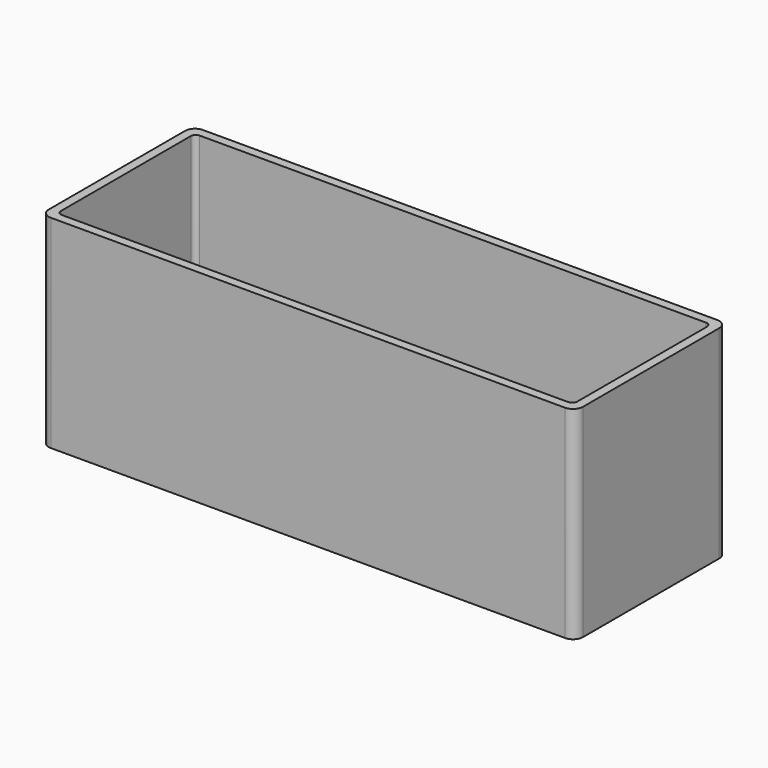
from build123d import *

# Parameters (mm, degrees)
F1_DEPTH = 40.64
F3_DEPTH = 38.608
F5_DEPTH = 4.7752
F6_R     = 1.35255
F7_DEPTH = 4.7752


# Not quite as in the source:
# - a feature names something its author has since deleted; it is built from what else it names


with BuildPart() as f1:
    # F0 (on Top) → F1 (new body)
    with BuildSketch(Plane.XY):
        with BuildLine():
            ThreePointArc((0, 2), (0.5857864376, 0.5857864376), (2, 0))
            Line((2, 0), (105.061, 0))
            ThreePointArc((105.061, 0), (106.4752135624, 0.5857864376), (107.061, 2))
            Line((107.061, 2), (107.061, 36.1))
            ThreePointArc((107.061, 36.1), (106.4752135624, 37.5142135624), (105.061, 38.1))
            Line((105.061, 38.1), (2, 38.1))
            ThreePointArc((2, 38.1), (0.5857864376, 37.5142135624), (0, 36.1))
            Line((0, 36.1), (0, 2))
        make_face()
    extrude(amount=F1_DEPTH)

    # F2 (on face) → F3 (cut)
    with BuildSketch(Plane.XY.offset(40.64)):
        with BuildLine():
            Line((104.261, 36.3), (2.8, 36.3))
            ThreePointArc((2.8, 36.3), (2.0928932188, 36.0071067812), (1.8, 35.3))
            Line((1.8, 35.3), (1.8, 2.8))
            ThreePointArc((1.8, 2.8), (2.0928932188, 2.0928932188), (2.8, 1.8))
            Line((2.8, 1.8), (104.261, 1.8))
            ThreePointArc((104.261, 1.8), (104.9681067812, 2.0928932188), (105.261, 2.8))
            Line((105.261, 2.8), (105.261, 35.3))
            ThreePointArc((105.261, 35.3), (104.9681067812, 36.0071067812), (104.261, 36.3))
        make_face()
    extrude(amount=-F3_DEPTH, mode=Mode.SUBTRACT)

    # F4 (on face) → F5 (join)
    with BuildSketch(Plane(origin=(0, 0, 0), x_dir=(1, 0, 0), z_dir=(0, 0, -1))):
        with BuildLine():
            ThreePointArc((107.061, -2), (106.4752135624, -0.5857864376), (105.061, 0))
            Line((105.061, 0), (101.251, 0))
            Line((101.251, 0), (101.251, -2))
            ThreePointArc((101.251, -2), (102.3669231637, -4.6940768363), (105.061, -5.81))
            Line((105.061, -5.81), (107.061, -5.81))
            Line((107.061, -5.81), (107.061, -2))
        make_face()
        with BuildLine():
            Line((101.251, -36.1), (101.251, -38.1))
            Line((101.251, -38.1), (105.061, -38.1))
            ThreePointArc((105.061, -38.1), (106.4752135624, -37.5142135624), (107.061, -36.1))
            Line((107.061, -36.1), (107.061, -32.29))
            Line((107.061, -32.29), (105.061, -32.29))
            ThreePointArc((105.061, -32.29), (102.3669231637, -33.4059231637), (101.251, -36.1))
        make_face()
        with BuildLine():
            ThreePointArc((5.81, -36.1), (4.6940768363, -33.4059231637), (2, -32.29))
            Line((2, -32.29), (0, -32.29))
            Line((0, -32.29), (0, -36.1))
            ThreePointArc((0, -36.1), (0.5857864376, -37.5142135624), (2, -38.1))
            Line((2, -38.1), (5.81, -38.1))
            Line((5.81, -38.1), (5.81, -36.1))
        make_face()
        with BuildLine():
            Line((5.81, 0), (2, 0))
            ThreePointArc((2, 0), (0.5857864376, -0.5857864376), (0, -2))
            Line((0, -2), (0, -5.81))
            Line((0, -5.81), (2, -5.81))
            ThreePointArc((2, -5.81), (4.6940768363, -4.6940768363), (5.81, -2))
            Line((5.81, -2), (5.81, 0))
        make_face()
    extrude(amount=-F5_DEPTH)

    # F6 (on face) → F7 (cut, through all)
    with BuildSketch(Plane(origin=(0, 0, 0), x_dir=(1, 0, 0), z_dir=(0, 0, -1))):
        with Locations((103.8037641431, -3.2572358569)):
            Circle(F6_R)
        with Locations((3.2572358569, -3.2572358569)):
            Circle(F6_R)
        with Locations((3.2572358569, -34.8427641431)):
            Circle(F6_R)
        with Locations((103.8037641431, -34.8427641431)):
            Circle(F6_R)
    extrude(amount=-F7_DEPTH, mode=Mode.SUBTRACT)


solid = f1.part
